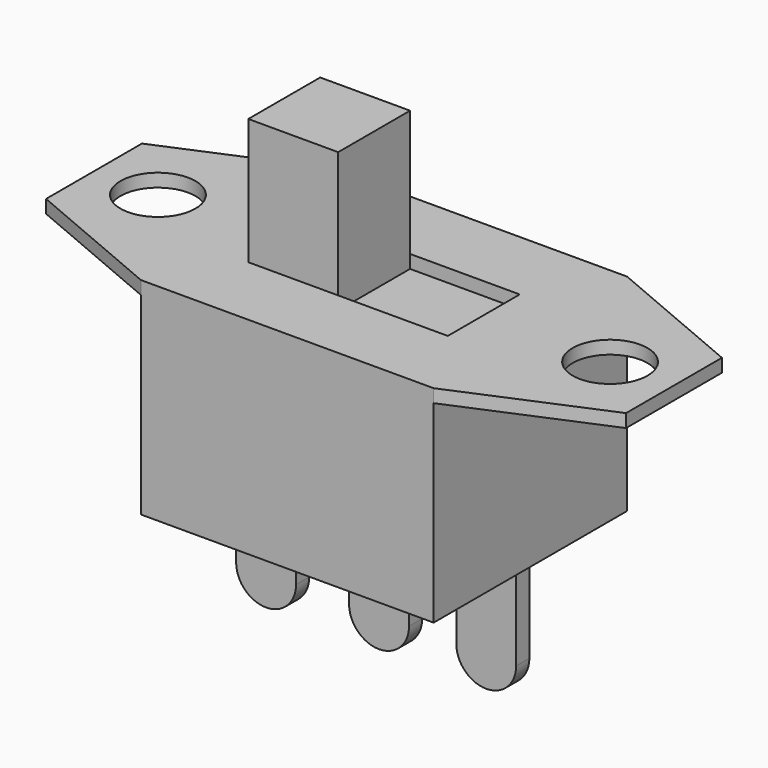
from build123d import *

# Parameters (mm, degrees)
F0_W     = 3
F0_H     = 3
F1_DEPTH = 4.65
F0_W_2   = 9.77
F0_H_2   = 8.07
F0_W_3   = 3.66
F2_DEPTH = 6.45
F0_R     = 1.25
F3_DEPTH = 0.44
F4_W     = 2
F4_H     = 0.55
F5_DEPTH = 3.88
F6_R     = 0.99999


# Not quite as in the source:
# - a fillet or chamfer is up to 0.001 mm smaller than in the source, because OpenCascade refuses the exact size


with BuildPart() as f1:
    # F0 (on Top) → F1 (new body)
    with BuildSketch(Plane.XY):
        with Locations((-1.83, 0)):
            Rectangle(F0_W, F0_H)
    extrude(amount=F1_DEPTH)

    # F0 (on Top) → F2 (join)
    with BuildSketch(Plane.XY):
        Rectangle(F0_W_2, F0_H_2)
        Polygon((-3.33, -1.5), (-3.33, 1.5), (-0.33, 1.5), (3.33, 1.5), (3.33, -1.5), (-0.33, -1.5), align=None, mode=Mode.SUBTRACT)
        with Locations((1.5, 0)):
            Rectangle(F0_W_3, F0_H)
        with Locations((-1.83, 0)):
            Rectangle(F0_W, F0_H)
    extrude(amount=-F2_DEPTH)

    # F0 (on Top) → F3 (join)
    with BuildSketch(Plane.XY):
        Polygon((-4.885, -4.035), (-4.885, 4.035), (-9.68, 2), (-9.68, -2), align=None)
        with Locations((-7.5463647954, 0)):
            Circle(F0_R, mode=Mode.SUBTRACT)
        Rectangle(F0_W_2, F0_H_2)
        Polygon((-3.33, -1.5), (-3.33, 1.5), (-0.33, 1.5), (3.33, 1.5), (3.33, -1.5), (-0.33, -1.5), align=None, mode=Mode.SUBTRACT)
        Polygon((9.68, 2), (4.885, 4.035), (4.885, -4.035), (9.68, -2), align=None)
        with Locations((7.5463647954, 0)):
            Circle(F0_R, mode=Mode.SUBTRACT)
    extrude(amount=F3_DEPTH)

    # F4 (on face) → F5 (join)
    with BuildSketch(Plane(origin=(0, 0, -6.45), x_dir=(1, 0, 0), z_dir=(0, 0, -1))):
        with Locations((-3.7156233341, 0)):
            Rectangle(F4_W, F4_H)
        with Locations((0.0545115434, 0)):
            Rectangle(F4_W, F4_H)
        with Locations((3.6328930184, 0)):
            Rectangle(F4_W, F4_H)
    extrude(amount=F5_DEPTH)

    # F6 (radius 1 in the source; OpenCascade refuses exactly that, so slightly less here)
    f6_edges = [f1.edges().sort_by_distance(p)[0] for p in [
        (-2.715623, 0, -10.33),
        (-4.715623, 0, -10.33),
        (-0.945488, 0, -10.33),
        (1.054512, 0, -10.33),
        (2.632893, 0, -10.33),
        (4.632893, 0, -10.33),
    ]]
    fillet(f6_edges, radius=F6_R)


solid = f1.part
